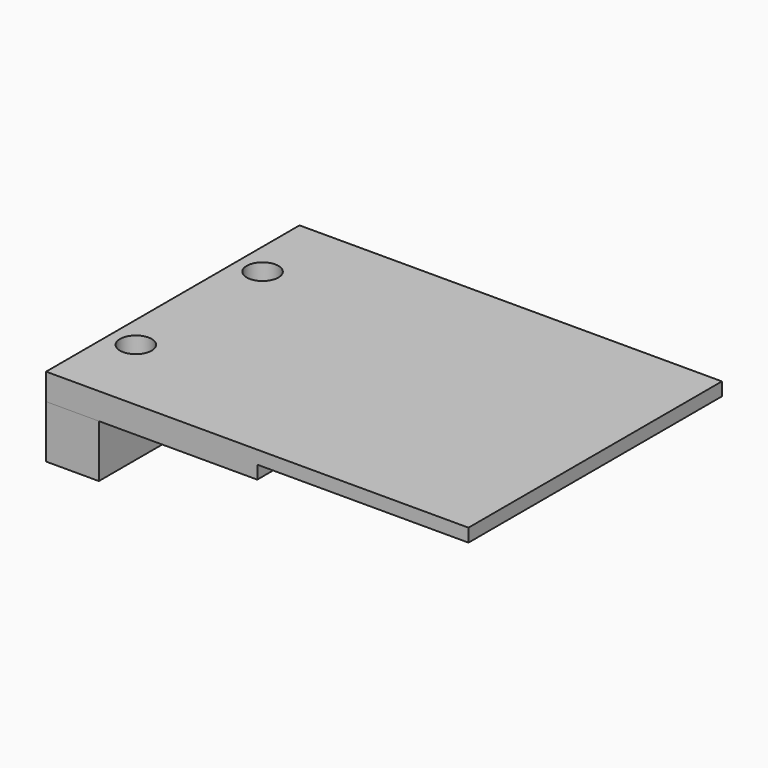
from build123d import *
from build123d import SkipClean  # not in build123d's __all__

# Parameters (mm, degrees)
F0_W     = 50.8
F0_H     = 3.175
F1_DEPTH = 76.2
F3_DEPTH = 6.351
F4_W     = 12.7
F4_H     = 76.2
F4_R     = 3.81
F5_DEPTH = 12.7


with BuildPart() as f1:
    # F0 (on Front) → F1 (new body)
    with BuildSketch(Plane.XZ):
        Polygon((25.4, 3.175), (-25.4, 3.175), (-25.4, -3.175), (25.4, -3.175), (25.4, 0), align=None)
        with Locations((50.8, 1.5875)):
            Rectangle(F0_W, F0_H)
    extrude(amount=F1_DEPTH)

    # F2 (on face) → F3 (cut, through all)
    with BuildSketch(Plane.XY.offset(3.175)):
        with BuildLine():
            Line((-22.86, -19.05), (-15.24, -19.05))
            ThreePointArc((-15.24, -19.05), (-19.05, -15.24), (-22.86, -19.05))
        make_face()
        with BuildLine():
            ThreePointArc((-22.86, -19.05), (-19.05, -22.86), (-15.24, -19.05))
            Line((-15.24, -19.05), (-22.86, -19.05))
        make_face()
        with BuildLine():
            Line((-22.86, -57.15), (-15.24, -57.15))
            ThreePointArc((-15.24, -57.15), (-19.05, -53.34), (-22.86, -57.15))
        make_face()
        with BuildLine():
            ThreePointArc((-22.86, -57.15), (-19.05, -60.96), (-15.24, -57.15))
            Line((-15.24, -57.15), (-22.86, -57.15))
        make_face()
    extrude(amount=-F3_DEPTH, mode=Mode.SUBTRACT)

    # F4 (on face) → F5 (join)
    with BuildSketch(Plane(origin=(0, 0, -3.175), x_dir=(1, 0, 0), z_dir=(0, 0, -1))):
        with Locations((-19.05, 38.1)):
            Rectangle(F4_W, F4_H)
        with Locations((-19.05, 19.05)):
            Circle(F4_R, mode=Mode.SUBTRACT)
        with Locations((-19.05, 57.15)):
            Circle(F4_R, mode=Mode.SUBTRACT)
    with SkipClean():  # cleaning this boolean's faces spoils the solid; the shape is the same uncleaned
        extrude(amount=F5_DEPTH)


solid = f1.part
